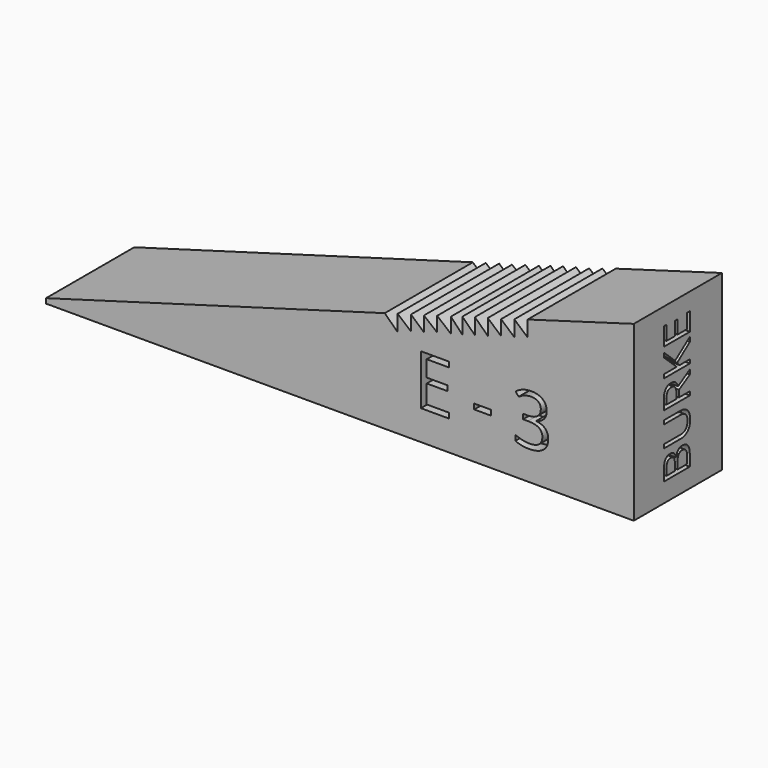
from build123d import *

# Parameters (mm, degrees)
F1_DEPTH     = 25
F2_TEXT_SIZE = 15.9423552557
F4_DEPTH     = 3
F3_TEXT_SIZE = 15.9423552557
F5_DEPTH     = 3
F6_TEXT_SIZE = 10.3319277838
F7_DEPTH     = 2


# Not quite as in the source:
# - Text() gives the source's letters only with a copy of the font that has no kerning and outlines rounded to 1/6400 em; it was checked with that copy


with BuildPart() as f1:
    # F0 (on Front) → F1 (new body)
    with BuildSketch(Plane.XZ):
        Polygon((-59.0122230351, -21.3820207864), (-57.9569935799, -21.3575270027), (74.3279606104, -21.3575270027), (74.3279606104, 17.9704297334), (50.2419397235, 11.0080651939), (50.2419397235, 7.432796061), (47.231182456, 10.0672040135), (47.231182456, 6.4919358119), (44.2204326391, 9.1263446957), (44.2204326391, 5.7392474264), (41.2096790969, 8.3736563101), (41.2096790969, 4.7983871773), (38.2793433964, 7.5989789329), (38.2793433964, 3.9946706966), (35.4294255376, 6.760767661), (35.4294255376, 3.1564596575), (32.8309722245, 5.9225563891), (32.8309722245, 2.4858908728), (29.7295898199, 5.0843455829), (29.7295898199, 1.7315007281), (26.7120301723, 4.1623134166), (26.7120301723, 0.8094683872), (23.7782914191, 3.407923039), (23.7782914191, 0), (20.7607299089, 2.569712), (20.7607299089, -1.11841748), (17.8269911557, 1.7315007281), (-59.0122230351, -20.2563684704), align=None)
    extrude(amount=F1_DEPTH)

    # F2 (on face) → F4 (cut)
    with BuildSketch(Plane.XZ.offset(25)):
        with Locations((24.4623702019, -14.5833347924)):
            Text('E - 3', F2_TEXT_SIZE, font='Open Sans', text_align=(TextAlign.LEFT, TextAlign.BOTTOM))
    extrude(amount=-F4_DEPTH, mode=Mode.SUBTRACT)

    # F3 (on face) → F5 (cut)
    with BuildSketch(Plane(origin=(0, 0, 0), x_dir=(-1, 0, 0), z_dir=(0, 1, 0))):
        with Locations((-55.9475468472, -14.8470071144)):
            Text('E - 3', F3_TEXT_SIZE, font='Open Sans', text_align=(TextAlign.LEFT, TextAlign.BOTTOM))
    extrude(amount=-F5_DEPTH, mode=Mode.SUBTRACT)

    # F6 (on face) → F7 (cut)
    with BuildSketch(Plane.YZ.offset(74.3279606104)):
        with Locations(Location((-9.1111809015, -18.0352659372), (0, 0, 90))):
            Text('BURKE', F6_TEXT_SIZE, font='Open Sans', text_align=(TextAlign.LEFT, TextAlign.BOTTOM))
    extrude(amount=-F7_DEPTH, mode=Mode.SUBTRACT)


solid = f1.part
